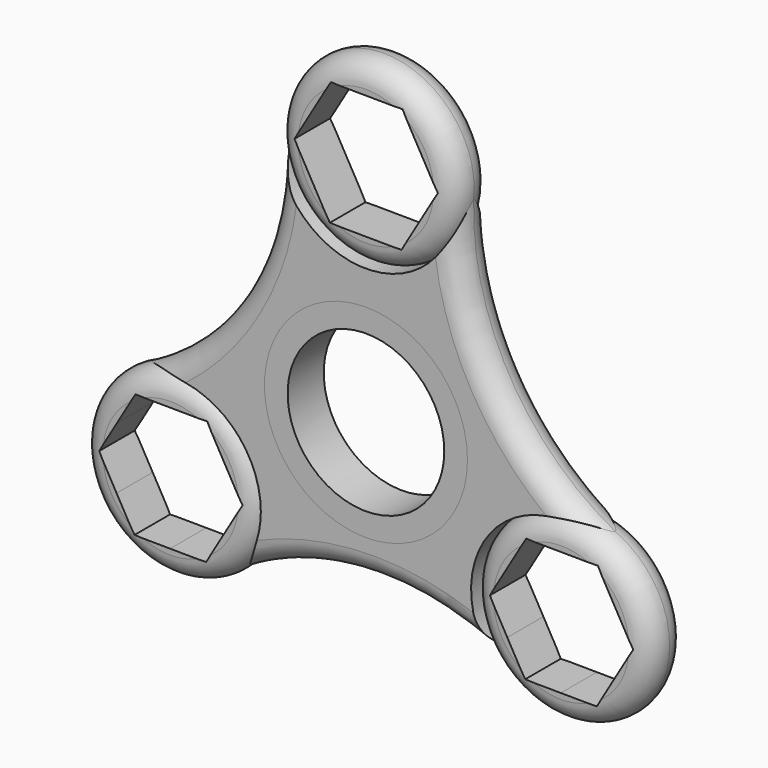
from build123d import *

# Parameters (mm, degrees)
F1_R     = 12.7
F4_DEPTH = 6.35
F2_R     = 14.2875
F0_R     = 12.7
F0_R_2   = 14.2875
F0_R_3   = 11.0236
F5_F1_R  = 3.175
F5_F2_R  = 3.175
F5_F3_R  = 3.175
F6_F1_R  = 3.1749
F6_F2_R  = 3.1749
F6_F3_R  = 3.1749


# Not quite as in the source:
# - a fillet or chamfer that OpenCascade refuses, or shapes differently, is made with other operations: its cross-section is extruded or revolved along the edge and cut away or added
# - a fillet or chamfer is up to 0.001 mm smaller than in the source, because OpenCascade refuses the exact size


with BuildPart() as f4:
    # F1 (on Front) → F4 (new body)
    with BuildSketch(Plane.XZ):
        with Locations((-27.4963065702, -15.875)):
            Circle(F1_R)
        Polygon((-22.3808230927, -7.1786769951), (-19.8940756321, -11.5678270844), (-17.4073281897, -15.9569771417), (-19.9650698809, -20.3051385633), (-22.5228116671, -24.6533001465), (-27.5673012489, -24.6123115725), (-32.6117900476, -24.5713230049), (-35.0985376675, -20.1821726344), (-37.5852849506, -15.7930228583), (-35.0275432594, -11.4448614367), (-32.4698014732, -7.0966998535), (-27.4253121544, -7.1376884253), align=None, mode=Mode.SUBTRACT)
    extrude(amount=F4_DEPTH)

    # F5#2: fillet of radius 3.175 on 1 edges, made by hand

    # F5_2_s1 → F5_2_t2 (revolve, cut)
    with BuildSketch(Plane.XY.offset(-15.875)):
        with BuildLine():
            ThreePointArc((-14.7963065702, -3.175), (-15.7262425399, -5.4200640303), (-17.9713065702, -6.35))
            Line((-17.9713065702, -6.35), (-14.7963065702, -6.35))
            Line((-14.7963065702, -6.35), (-14.7963065702, -3.175))
        make_face()
    revolve(axis=Axis((-27.4963065702, -6.35, -15.875), (0, -1, 0)), mode=Mode.SUBTRACT)

    # F6#3: fillet of radius 3.175 on 1 edges, made by hand

    # F6_3_s1 → F6_3_t2 (revolve, cut)
    with BuildSketch(Plane.XY.offset(-15.875)):
        with BuildLine():
            ThreePointArc((-14.7963065702, -3.175), (-15.7262425399, -0.9299359697), (-17.9713065702, 0))
            Line((-17.9713065702, 0), (-14.7963065702, 0))
            Line((-14.7963065702, 0), (-14.7963065702, -3.175))
        make_face()
    revolve(axis=Axis((-27.4963065702, 0, -15.875), (0, -1, 0)), mode=Mode.SUBTRACT)


with BuildPart() as f4b:
    # F1 (on Front) → F4, piece 2 (new body)
    with BuildSketch(Plane.XZ):
        with Locations((27.4963065702, -15.875)):
            Circle(F1_R)
        Polygon((32.6117900476, -7.1786769951), (35.0985372903, -11.5678266998), (37.5852849506, -15.9569771417), (35.0275432594, -20.3051385633), (32.4698014732, -24.6533001465), (27.4253122046, -24.6123115751), (22.3808230927, -24.5713230049), (19.8940755771, -20.1821728184), (17.4073281897, -15.7930228583), (19.9650701204, -11.4448610295), (22.5228116671, -7.0966998535), (27.5673012991, -7.1376884279), align=None, mode=Mode.SUBTRACT)
    extrude(amount=F4_DEPTH)

    # F5#3: fillet of radius 3.175 on 1 edges, made by hand

    # F5_3_s1 → F5_3_t2 (revolve, cut)
    with BuildSketch(Plane.XY.offset(-15.875)):
        with BuildLine():
            ThreePointArc((40.1963065702, -3.175), (39.2663706004, -5.4200640303), (37.0213065702, -6.35))
            Line((37.0213065702, -6.35), (40.1963065702, -6.35))
            Line((40.1963065702, -6.35), (40.1963065702, -3.175))
        make_face()
    revolve(axis=Axis((27.4963065702, -6.35, -15.875), (0, -1, 0)), mode=Mode.SUBTRACT)

    # F6#2: fillet of radius 3.175 on 1 edges, made by hand

    # F6_2_s1 → F6_2_t2 (revolve, cut)
    with BuildSketch(Plane.XY.offset(-15.875)):
        with BuildLine():
            ThreePointArc((40.1963065702, -3.175), (39.2663706004, -0.9299359697), (37.0213065702, 0))
            Line((37.0213065702, 0), (40.1963065702, 0))
            Line((40.1963065702, 0), (40.1963065702, -3.175))
        make_face()
    revolve(axis=Axis((27.4963065702, 0, -15.875), (0, -1, 0)), mode=Mode.SUBTRACT)


with BuildPart() as f4c:
    # F2 (on Front) → F4, piece 3 (new body)
    with BuildSketch(Plane.XZ):
        with BuildLine():
            ThreePointArc((-32.4698014732, -4.189352887), (-20.4917860751, -5.2812899495), (-14.7963065702, -15.875))
            ThreePointArc((-14.7963065702, -15.875), (-15.7397207314, -20.6784039405), (-18.4298009663, -24.768170196))
            ThreePointArc((-18.4298009663, -24.768170196), (-1.0309003528, -19.4158776432), (16.8542129011, -22.8057894455))
            ThreePointArc((16.8542129011, -22.8057894455), (17.7865075947, -7.6890483842), (32.5279818117, -4.2142862884))
            ThreePointArc((32.5279818117, -4.2142862884), (17.6527755106, 10.2318394169), (12.622369648, 30.3479356399))
            ThreePointArc((12.622369648, 30.3479356399), (0.0015548934, 19.0500000952), (-12.6220259529, 30.344844904))
            ThreePointArc((-12.6220259529, 30.344844904), (-17.6352111398, 10.2554270159), (-32.4698014732, -4.189352887))
        make_face()
        Circle(F2_R, mode=Mode.SUBTRACT)
    extrude(amount=F4_DEPTH)

    # F5: fillet of radius 3.175 on 3 edges, made by hand

    # F5_f1
    f5_f1_edges = [f4c.edges().sort_by_distance(p)[0] for p in [
        (-1.0309003528, -6.35, -19.4158776432),
    ]]
    fillet(f5_f1_edges, radius=F5_F1_R)

    # F5_f2
    f5_f2_edges = [f4c.edges().sort_by_distance(p)[0] for p in [
        (17.6527755106, -6.35, 10.2318394169),
    ]]
    fillet(f5_f2_edges, radius=F5_F2_R)

    # F5_f3
    f5_f3_edges = [f4c.edges().sort_by_distance(p)[0] for p in [
        (-17.6352111398, -6.35, 10.2554270159),
    ]]
    fillet(f5_f3_edges, radius=F5_F3_R)

    # F6: fillet of radius 3.175 on 3 edges, made by hand

    # F6_f1 (radius 3.175 in the source; OpenCascade refuses exactly that, so slightly less here)
    f6_f1_edges = [f4c.edges().sort_by_distance(p)[0] for p in [
        (-1.0309003528, 0, -19.4158776432),
    ]]
    fillet(f6_f1_edges, radius=F6_F1_R)

    # F6_f2 (radius 3.175 in the source; OpenCascade refuses exactly that, so slightly less here)
    f6_f2_edges = [f4c.edges().sort_by_distance(p)[0] for p in [
        (-17.6352111398, 0, 10.2554270159),
    ]]
    fillet(f6_f2_edges, radius=F6_F2_R)

    # F6_f3 (radius 3.175 in the source; OpenCascade refuses exactly that, so slightly less here)
    f6_f3_edges = [f4c.edges().sort_by_distance(p)[0] for p in [
        (17.6527755106, 0, 10.2318394169),
    ]]
    fillet(f6_f3_edges, radius=F6_F3_R)


with BuildPart() as f4d:
    # F0 (on Front) → F4, piece 4 (new body)
    with BuildSketch(Plane.XZ):
        with Locations((0, 31.75)):
            Circle(F0_R)
        Polygon((5.1154834774, 40.4463230049), (10.0889783805, 31.6680228583), (4.973494903, 22.9716998535), (-5.1154834774, 23.0536769951), (-10.0889783805, 31.8319771417), (-4.973494903, 40.5283001465), align=None, mode=Mode.SUBTRACT)
    extrude(amount=F4_DEPTH)

    # F5#4: fillet of radius 3.175 on 1 edges, made by hand

    # F5_4_s1 → F5_4_t2 (revolve, cut)
    with BuildSketch(Plane.XY.offset(31.75)):
        with BuildLine():
            ThreePointArc((12.7, -3.175), (11.7700640303, -5.4200640303), (9.525, -6.35))
            Line((9.525, -6.35), (12.7, -6.35))
            Line((12.7, -6.35), (12.7, -3.175))
        make_face()
    revolve(axis=Axis((0, -6.35, 31.75), (0, -1, 0)), mode=Mode.SUBTRACT)

    # F6#4: fillet of radius 3.175 on 1 edges, made by hand

    # F6_4_s1 → F6_4_t2 (revolve, cut)
    with BuildSketch(Plane.XY.offset(31.75)):
        with BuildLine():
            ThreePointArc((12.7, -3.175), (11.7700640303, -0.9299359697), (9.525, 0))
            Line((9.525, 0), (12.7, 0))
            Line((12.7, 0), (12.7, -3.175))
        make_face()
    revolve(axis=Axis((0, 0, 31.75), (0, -1, 0)), mode=Mode.SUBTRACT)


with BuildPart() as f4e:
    # F0 (on Front) → F4, piece 5 (new body)
    with BuildSketch(Plane.XZ):
        Circle(F0_R_2)
        Circle(F0_R_3, mode=Mode.SUBTRACT)
    extrude(amount=F4_DEPTH)


solid = Compound([f4.part, f4b.part, f4c.part, f4d.part, f4e.part])
